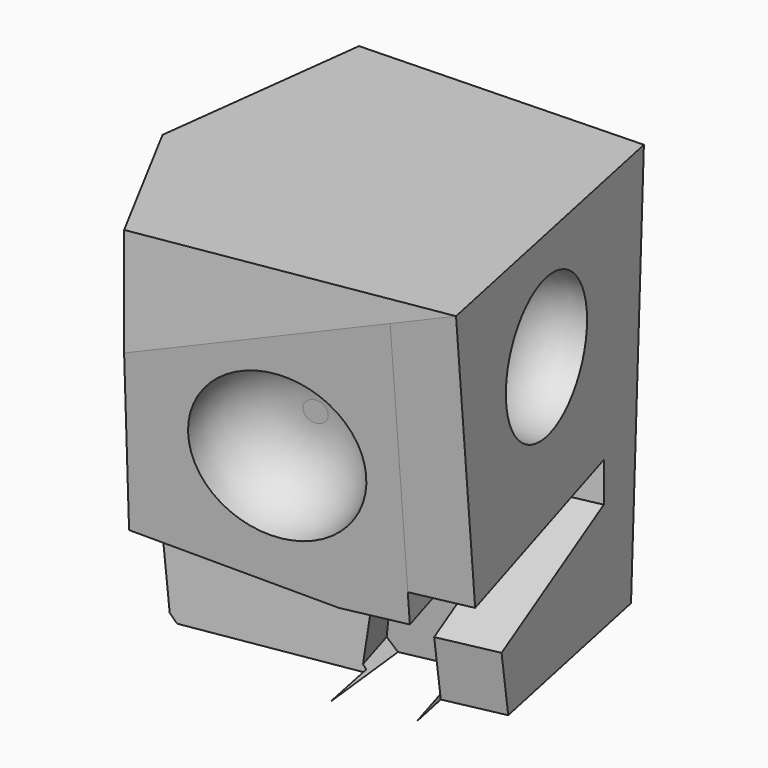
from build123d import *

# Parameters (mm, degrees)
F1_DEPTH  = 100
F6_DEPTH  = 25
F7_DEPTH  = 15
F9_DEPTH  = 25
F3_R      = 17.8601151659
F10_DEPTH = 13
F11_R     = 12.99999
F13_DEPTH = 25
F14_DEPTH = 90
F12_R     = 19.8108840593
F15_DEPTH = 17
F16_R     = 16.99999
F18_DEPTH = 25


# Not quite as in the source:
# - a fillet or chamfer is up to 0.001 mm smaller than in the source, because OpenCascade refuses the exact size


with BuildPart() as f1:
    # F0 (on Top) → F1 (new body)
    with BuildSketch(Plane.XY):
        Polygon((-47.5200526416, -19.4592215121), (-27.9358569533, -56.1545789242), (46.7044450343, -43.9518280327), (29.7740362585, 36.9222164154), (-40.8926419914, 34.7126610577), align=None)
    extrude(amount=F1_DEPTH)

    # F5 (on 3pt) → F6 (cut)
    with BuildSketch(Plane(origin=(9.6412332648, 36.848921293, -1.9307798529), x_dir=(0.9675193136, -0.2524507981, 0.0132277119), z_dir=(-0.2527971081, -0.9661938968, 0.0506258432))):
        Polygon((22.0081010682, 1.6419123086), (20.808683311, 101.7949787998), (2.3196212658, 1.9027031079), align=None)
    extrude(amount=-F6_DEPTH, mode=Mode.SUBTRACT)

    # F3 (on face) → F7 (cut)
    with BuildSketch(Plane(origin=(35.9288773181, 7.5214561607, 0), x_dir=(-0.2049012214, 0.9787826569, 0), z_dir=(0.9787826569, 0.2049012214, 0))):
        Polygon((-44.1726371646, 30.7864621282), (-52.589084849, 100), (-52.589084849, 0), (-29.6385996044, 0), (-32.5648710132, 15.3381312266), (12.4055901776, 27.6119541377), (12.4055901776, 37.6664411777), align=None)
    extrude(amount=-F7_DEPTH, mode=Mode.SUBTRACT)

    # F8 (on face) → F9 (cut)
    with BuildSketch(Plane(origin=(8.1632362237, -38.9945652191, -4.8445740248), x_dir=(0.979095124, 0.2018510885, 0.0250774059), z_dir=(0.2034028962, -0.9716253806, -0.1207119775))):
        Polygon((39.3641106636, 104.6558680882), (-79.5409610954, 107.6664552623), (-81.3024698416, 37.9594929491), (22.60753629, 35.3336665102), (24.2297143871, 99.5269938077), align=None)
        Polygon((22.60753629, 35.3336665102), (-81.3024698416, 37.9594929491), (-82.4683913698, -8.1787100022), (37.6027492107, -11.21293151), (37.6027492107, 34.9547345092), align=None)
    extrude(amount=F9_DEPTH, mode=Mode.SUBTRACT)

    # F3 (on face) → F10 (cut)
    with BuildSketch(Plane(origin=(35.9288773181, 7.5214561607, 0), x_dir=(-0.2049012214, 0.9787826569, 0), z_dir=(0.9787826569, 0.2049012214, 0))):
        with Locations((-12.8240771592, 72.3933577538)):
            Circle(F3_R)
    extrude(amount=-F10_DEPTH, mode=Mode.SUBTRACT)

    # F11 (radius 13 in the source; OpenCascade refuses exactly that, so slightly less here)
    f11_edges = [f1.edges().sort_by_distance(p)[0] for p in [
        (29.491931, -25.175415, 72.393358),
    ]]
    fillet(f11_edges, radius=F11_R)

    # F12 (on face) → F13 (cut)
    with BuildSketch(Plane(origin=(8.1632362237, -38.9945652191, -4.8445740248), x_dir=(0.979095124, 0.2018510885, 0.0250774059), z_dir=(0.2034028962, -0.9716253806, -0.1207119775))):
        Polygon((21.8240755779, 4.3303198355), (22.4123828022, 27.6109930646), (6.6332079808, 28.009735938), (2.6960770767, 4.8136881468), align=None)
        Polygon((18.9769355737, -4.4831562801), (21.8240755779, 4.3303198355), (2.6960770767, 4.8136881468), (9.4391942611, -4.4458445128), align=None)
    extrude(amount=-F13_DEPTH, mode=Mode.SUBTRACT)

    # F12 (on face) → F14 (cut)
    with BuildSketch(Plane(origin=(8.1632362237, -38.9945652191, -4.8445740248), x_dir=(0.979095124, 0.2018510885, 0.0250774059), z_dir=(0.2034028962, -0.9716253806, -0.1207119775))):
        Polygon((-50.4545168754, 2.399114297), (-41.2831704405, 5.9250524436), (-47.9467762851, 101.636191148), align=None)
        Polygon((-33.0309979628, -4.2797005717), (-41.2831704405, 5.9250524436), (-50.4545168754, 2.399114297), align=None)
    extrude(amount=-F14_DEPTH, mode=Mode.SUBTRACT)

    # F12 (on face) → F15 (cut)
    with BuildSketch(Plane(origin=(8.1632362237, -38.9945652191, -4.8445740248), x_dir=(0.979095124, 0.2018510885, 0.0250774059), z_dir=(0.2034028962, -0.9716253806, -0.1207119775))):
        with Locations((-4.2161699384, 61.7149807513)):
            Circle(F12_R)
    extrude(amount=-F15_DEPTH, mode=Mode.SUBTRACT)

    # F16 (radius 17 in the source; OpenCascade refuses exactly that, so slightly less here)
    f16_edges = [f1.edges().sort_by_distance(p)[0] for p in [
        (-18.819384, -34.935619, 57.849136),
    ]]
    fillet(f16_edges, radius=F16_R)

    # F17 (on face) → F18 (cut)
    with BuildSketch(Plane(origin=(8.2143401196, -50.2444762342, 0), x_dir=(0.9868979975, 0.1613454139, 0), z_dir=(0.1613454139, -0.9868979975, 0))):
        Polygon((7.8329915962, 23.1178128028), (-44.1760422775, 30.926933164), (-42.148109545, 7.0275762015), (-39.5882407468, 0), (4.361868039, 0), align=None)
    extrude(amount=-F18_DEPTH, mode=Mode.SUBTRACT)


solid = f1.part
